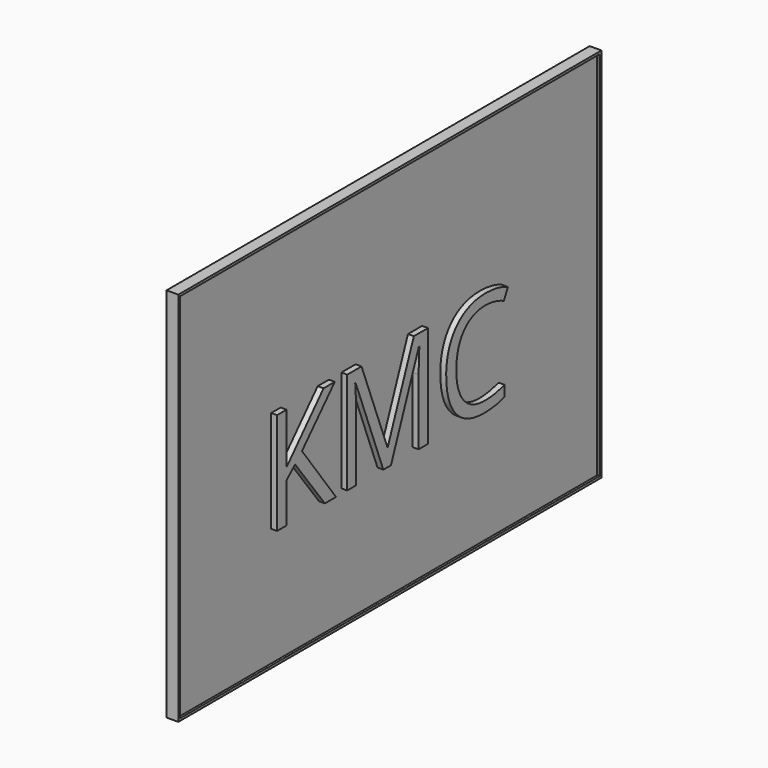
from build123d import *

# Parameters (mm, degrees)
F0_W         = 450
F0_H         = 320
F1_DEPTH     = 10
F2_W         = 446
F2_H         = 316
F3_DEPTH     = 2
F4_W         = 300
F4_H         = 200
F5_DEPTH     = 15
F6_R         = 5
F7_R         = 5
F8_DEPTH     = 8
F9_TEXT_SIZE = 121.5426632831
F10_DEPTH    = 5


# Not quite as in the source:
# - Text() gives the source's letters only with a copy of the font that has no kerning and outlines rounded to 1/6400 em; it was checked with that copy


with BuildPart() as f1:
    # F0 (on Right) → F1 (new body)
    with BuildSketch(Plane.YZ):
        with Locations((178.7242040038, 144.5743495971)):
            Rectangle(F0_W, F0_H)
    extrude(amount=F1_DEPTH)

    # F2 (on face) → F3 (cut)
    with BuildSketch(Plane.YZ.offset(10)):
        with Locations((178.7242040038, 144.5743495971)):
            Rectangle(F2_W, F2_H)
    extrude(amount=-F3_DEPTH, mode=Mode.SUBTRACT)

    # F4 (on face) → F5 (join)
    with BuildSketch(Plane(origin=(0, 0, 0), x_dir=(0, -1, 0), z_dir=(-1, 0, 0))):
        with Locations((-178.7242040038, 154.5743495971)):
            Rectangle(F4_W, F4_H)
    extrude(amount=F5_DEPTH)

    # F6
    f6_edges = [f1.edges().sort_by_distance(p)[0] for p in [
        (-15, 178.724204, 254.57435),
        (-15, 328.724204, 154.57435),
        (0, 178.724204, 254.57435),
        (0, 328.724204, 154.57435),
        (0, 178.724204, 54.57435),
        (0, 28.724204, 154.57435),
        (-15, 28.724204, 154.57435),
        (-7.5, 28.724204, 54.57435),
        (-15, 178.724204, 54.57435),
        (-7.5, 328.724204, 54.57435),
    ]]
    fillet(f6_edges, radius=F6_R)

    # F7 (on face) → F8 (join)
    with BuildSketch(Plane(origin=(-15, 0, 0), x_dir=(0, -1, 0), z_dir=(-1, 0, 0))):
        with Locations((-173.7242040038, 149.5743495971)):
            Circle(F7_R)
    extrude(amount=F8_DEPTH)

    # F9 (on face) → F10 (join)
    with BuildSketch(Plane.YZ.offset(8)):
        with Locations((43.0907726961, 87.3634535533)):
            Text('KMC', F9_TEXT_SIZE, font='Open Sans', text_align=(TextAlign.LEFT, TextAlign.BOTTOM))
    extrude(amount=F10_DEPTH)


solid = f1.part
